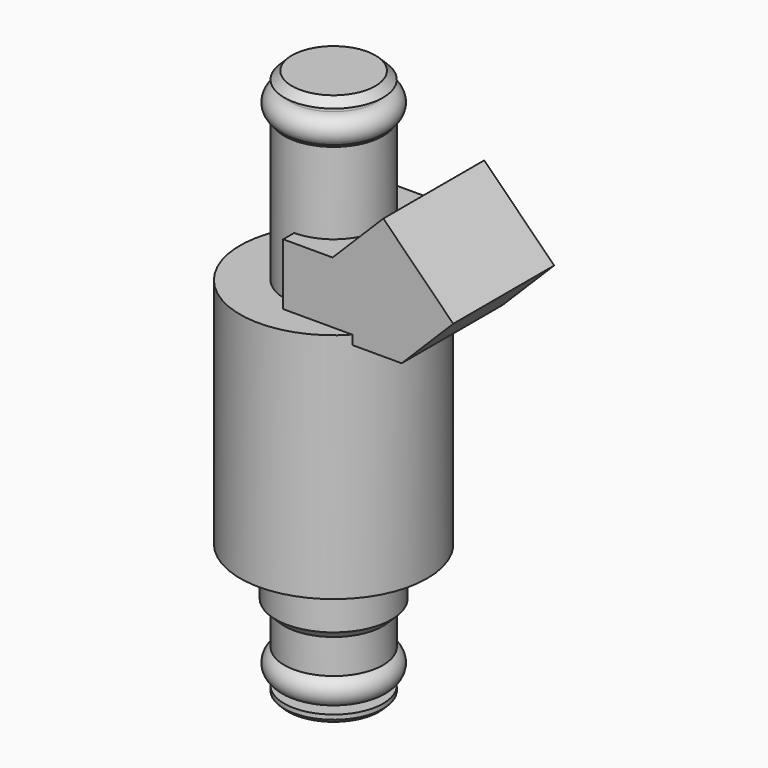
from build123d import *

# Parameters (mm, degrees)
F3_DEPTH = 8.3058


with BuildPart() as f1:
    # F0 (on Front) → F1 (revolve)
    with BuildSketch(Plane.XZ):
        with BuildLine():
            Line((5.4849602437, 72.39), (0, 72.39))
            Line((0, 72.39), (0, 0))
            Line((0, 0), (5.9791589156, 0))
            Line((5.9791589156, 0), (6.5, 0.5208410844))
            Line((6.5, 0.5208410844), (6.5, 1.1235540733))
            Line((6.5, 1.1235540733), (3.81, 1.1235540733))
            Line((3.81, 1.1235540733), (3.81, 1.958))
            Line((3.81, 1.958), (5.625, 1.958))
            ThreePointArc((5.625, 1.958), (7.44, 3.773), (5.625, 5.588))
            Line((5.625, 5.588), (6.5, 5.588))
            Line((6.5, 5.588), (6.5, 10.1114138961))
            Line((6.5, 10.1114138961), (7.62, 11.2314138961))
            Line((7.62, 11.2314138961), (7.62, 17.5331309438))
            Line((7.62, 17.5331309438), (12.319, 17.5331309438))
            Line((12.319, 17.5331309438), (12.319, 48.1258220971))
            Line((12.319, 48.1258220971), (6.5, 48.1258220971))
            Line((6.5, 48.1258220971), (6.5, 66.929))
            Line((6.5, 66.929), (5.625, 66.929))
            ThreePointArc((5.625, 66.929), (7.44, 68.744), (5.625, 70.559))
            Line((5.625, 70.559), (3.81, 70.559))
            Line((3.81, 70.559), (3.81, 71.3749602437))
            Line((3.81, 71.3749602437), (6.5, 71.3749602437))
            Line((6.5, 71.3749602437), (5.4849602437, 72.39))
        make_face()
    revolve(axis=Axis((0, 0, 36.195), (0, 0, -1)))

    # F2 (on Front) → F3 (join, symmetric)
    with BuildSketch(Plane.XZ):
        Polygon((13.188126497, 62.9115402699), (6.5, 56.2234137729), (0, 56.2234137729), (0, 46.9192864976), (12.319, 46.9192864976), (15.6018657007, 46.9192864976), (22.391122985, 53.7085437818), align=None)
    extrude(amount=F3_DEPTH, both=True)


solid = f1.part
